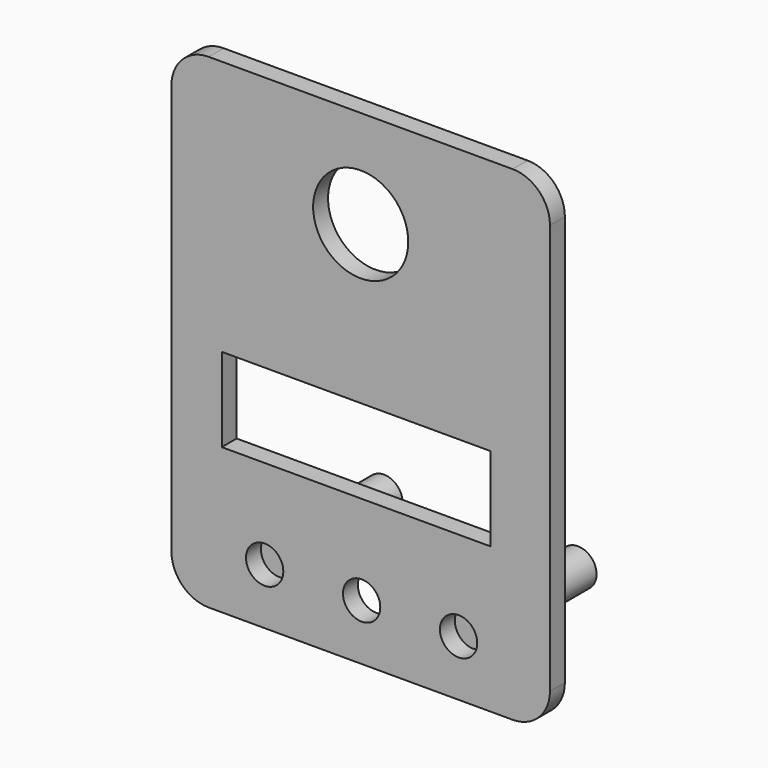
from build123d import *

# Parameters (mm, degrees)
F0_R     = 0.5
F0_W     = 7.2
F0_H     = 2.25
F0_R_2   = 1.275
F1_DEPTH = 0.5
F2_DEPTH = 3.5
F3_DEPTH = 1


# Not quite as in the source:
# - a feature names something its author has since deleted; it is built from what else it names


with BuildPart() as f1:
    # F0 (on Front) → F1 (new body)
    with BuildSketch(Plane.XZ):
        with BuildLine():
            ThreePointArc((-14.3548552409, -4.9672579244), (-15.0619620221, -5.2601511432), (-15.3548552409, -5.9672579244))
            Line((-15.3548552409, -5.9672579244), (-15.3548552409, -16.9672579244))
            ThreePointArc((-15.3548552409, -16.9672579244), (-15.0619620221, -17.6743647056), (-14.3548552409, -17.9672579244))
            Line((-14.3548552409, -17.9672579244), (-6.2048552409, -17.9672579244))
            ThreePointArc((-6.2048552409, -17.9672579244), (-5.4977484597, -17.6743647056), (-5.2048552409, -16.9672579244))
            Line((-5.2048552409, -16.9672579244), (-5.2048552409, -5.9672579244))
            ThreePointArc((-5.2048552409, -5.9672579244), (-5.4977484597, -5.2601511432), (-6.2048552409, -4.9672579244))
            Line((-6.2048552409, -4.9672579244), (-14.3548552409, -4.9672579244))
        make_face()
        with Locations((-12.8548552409, -16.4672579244)):
            Circle(F0_R, mode=Mode.SUBTRACT)
        with Locations((-10.4048552409, -12.9422579244)):
            Rectangle(F0_W, F0_H, mode=Mode.SUBTRACT)
        with Locations((-10.2548552409, -16.4672579244)):
            Circle(F0_R, mode=Mode.SUBTRACT)
        with Locations((-7.6548552409, -16.4672579244)):
            Circle(F0_R, mode=Mode.SUBTRACT)
        with Locations((-10.2798552409, -7.5972579244)):
            Circle(F0_R_2, mode=Mode.SUBTRACT)
    extrude(amount=F1_DEPTH)

    # F0 (on Front) → F3 (cut)
    with BuildSketch(Plane.XZ):
        with Locations((-10.4048552409, -12.9422579244)):
            Rectangle(F0_W, F0_H)
    extrude(amount=-F3_DEPTH, mode=Mode.SUBTRACT)


with BuildPart() as f2:
    # F0 (on Front) → F2 (new body)
    with BuildSketch(Plane.XZ):
        with Locations((-12.8548552409, -16.4672579244)):
            Circle(F0_R)
    extrude(amount=-F2_DEPTH)


with BuildPart() as f2b:
    # F0 (on Front) → F2, piece 2 (new body)
    with BuildSketch(Plane.XZ):
        with Locations((-7.6548552409, -16.4672579244)):
            Circle(F0_R)
    extrude(amount=-F2_DEPTH)


solid = Compound([f1.part, f2.part, f2b.part])
